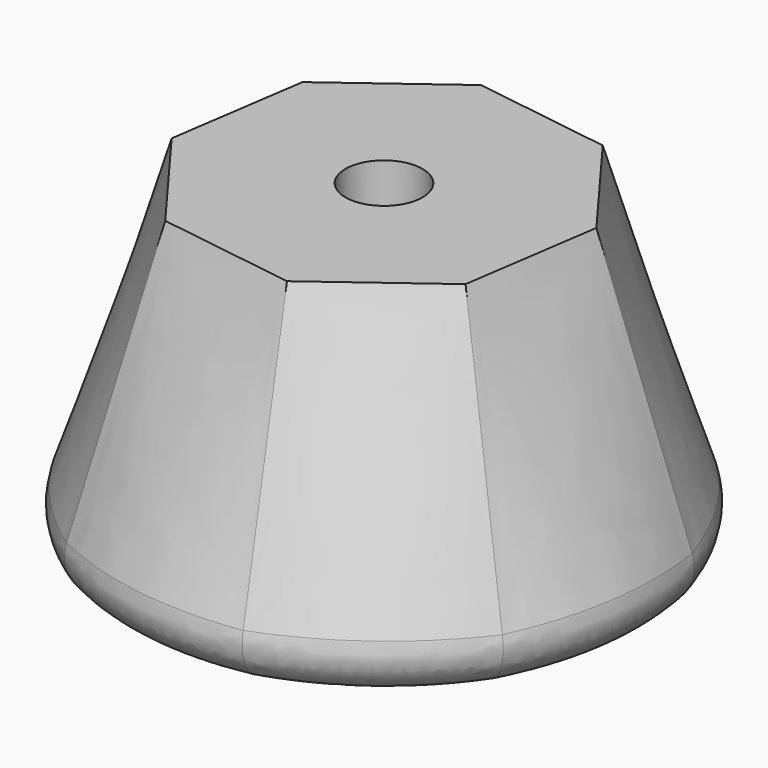
from build123d import *

# Parameters (mm, degrees)
F4_D     = 2.4
F4_DEPTH = 5
F4_TIP   = 0.7210327428
F5_R     = 1.27


# Not quite as in the source:
# - the arcs of a loft's sections are written as splines that run evenly, so that the points pair up as in the source's solid


with BuildPart() as f3:
    # F0 (on Top) → F3 section 0
    with BuildSketch(Plane.XY):
        with BuildLine():
            add(Edge.make_bspline(
                [(2.1287545667, -8.4725466174), (3.2378083255, -8.1938932963), (4.2910199355, -7.694831903), (6.1270120531, -6.3311147047), (6.9090701762, -5.4669954641), (7.4962519567, -4.4857383775)],
                knots=[0, 0, 0, 0, 0.5, 0.5, 1, 1, 1, 1], degree=3))
            add(Edge.make_bspline(
                [(7.4962519567, -4.4857383775), (8.0834337372, -3.504481291), (8.4752771134, -2.4068585241), (8.8092259113, -0.144322369), (8.7511999386, 1.0197008079), (8.4725466174, 2.1287545667)],
                knots=[0, 0, 0, 0, 0.5, 0.5, 1, 1, 1, 1], degree=3))
            add(Edge.make_bspline(
                [(8.4725466174, 2.1287545667), (8.1938932963, 3.2378083255), (7.694831903, 4.2910199355), (6.3311147047, 6.1270120531), (5.4669954641, 6.9090701762), (4.4857383775, 7.4962519567)],
                knots=[0, 0, 0, 0, 0.5, 0.5, 1, 1, 1, 1], degree=3))
            add(Edge.make_bspline(
                [(4.4857383775, 7.4962519567), (3.504481291, 8.0834337372), (2.4068585241, 8.4752771134), (0.144322369, 8.8092259113), (-1.0197008079, 8.7511999386), (-2.1287545667, 8.4725466174)],
                knots=[0, 0, 0, 0, 0.5, 0.5, 1, 1, 1, 1], degree=3))
            add(Edge.make_bspline(
                [(-2.1287545667, 8.4725466174), (-3.2378083255, 8.1938932963), (-4.2910199355, 7.694831903), (-6.1270120531, 6.3311147047), (-6.9090701762, 5.4669954641), (-7.4962519567, 4.4857383775)],
                knots=[0, 0, 0, 0, 0.5, 0.5, 1, 1, 1, 1], degree=3))
            add(Edge.make_bspline(
                [(-7.4962519567, 4.4857383775), (-8.0834337372, 3.504481291), (-8.4752771134, 2.4068585241), (-8.8092259113, 0.144322369), (-8.7511999386, -1.0197008079), (-8.4725466174, -2.1287545667)],
                knots=[0, 0, 0, 0, 0.5, 0.5, 1, 1, 1, 1], degree=3))
            add(Edge.make_bspline(
                [(-8.4725466174, -2.1287545667), (-8.1938932963, -3.2378083255), (-7.694831903, -4.2910199355), (-6.3311147047, -6.1270120531), (-5.4669954641, -6.9090701762), (-4.4857383775, -7.4962519567)],
                knots=[0, 0, 0, 0, 0.5, 0.5, 1, 1, 1, 1], degree=3))
            add(Edge.make_bspline(
                [(-4.4857383775, -7.4962519567), (-3.504481291, -8.0834337372), (-2.4068585241, -8.4752771134), (-0.144322369, -8.8092259113), (1.0197008079, -8.7511999386), (2.1287545667, -8.4725466174)],
                knots=[0, 0, 0, 0, 0.5, 0.5, 1, 1, 1, 1], degree=3))
        make_face()
    # F2 (on offset) → F3 section 1
    with BuildSketch(Plane.XY.offset(10)):
        Polygon((1.3828789294, -5.5039253369), (4.8697059974, -2.9140198603), (5.5039253369, 1.3828789294), (2.9140198603, 4.8697059974), (-1.3828789294, 5.5039253369), (-4.8697059974, 2.9140198603), (-5.5039253369, -1.3828789294), (-2.9140198603, -4.8697059974), align=None)
    loft(ruled=True)

    # F4
    with Locations(Plane.XY.offset(10)):
        with Locations((0, 0)):
            Hole(F4_D / 2, depth=F4_DEPTH)
            with Locations((0, 0, -(F4_DEPTH + F4_TIP / 2))):  # 118° drill point
                Cone(0, F4_D / 2, F4_TIP, mode=Mode.SUBTRACT)

    # F5
    f5_edges = [f3.edges().sort_by_distance(p)[0] for p in [
        (5.209016, -7.012973, 0),
        (8.642252, -1.27559, 0),
        (7.012973, 5.209016, 0),
        (1.27559, 8.642252, 0),
        (-5.209016, 7.012973, 0),
        (-8.642252, 1.27559, 0),
        (-7.012973, -5.209016, 0),
        (-1.27559, -8.642252, 0),
    ]]
    fillet(f5_edges, radius=F5_R)


solid = f3.part
